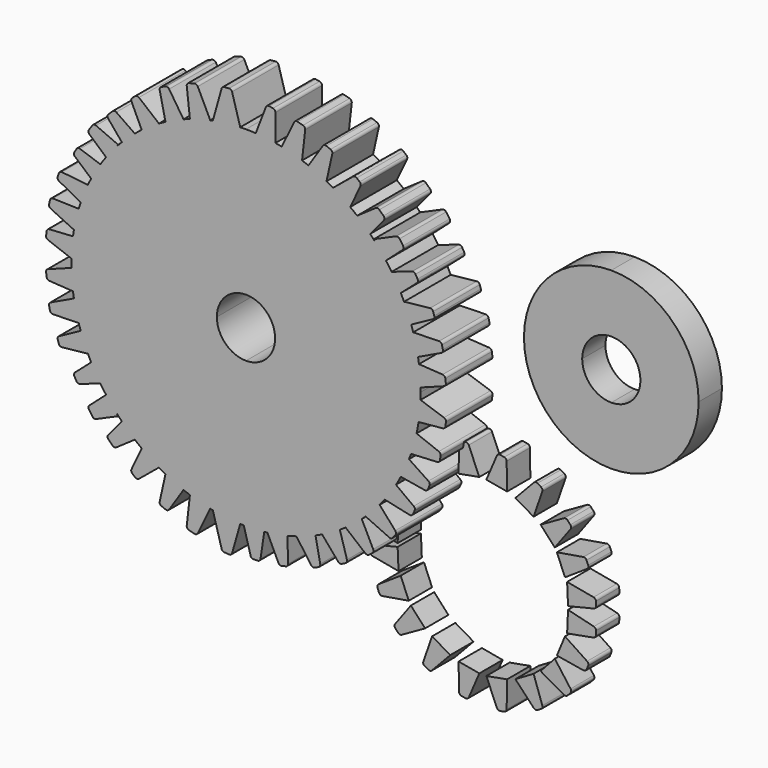
from build123d import *

# Parameters (mm, degrees)
F1_DEPTH = 12.7
F3_DEPTH = 6.35
F5_DEPTH = 12.7


with BuildPart() as f1:
    # F0 (on Front) → F1 (new body)
    with BuildSketch(Plane.XZ):
        with BuildLine():
            Line((-40.2337083757, 35.2117754519), (-8.4837083757, 35.2117754519))
            ThreePointArc((-8.4837083757, 35.2117754519), (-19.6429400125, 62.1525438151), (-46.5837083757, 73.3117754519))
            Line((-46.5837083757, 73.3117754519), (-46.5837083757, 41.5617754519))
            ThreePointArc((-46.5837083757, 41.5617754519), (-42.0935803152, 39.7019035124), (-40.2337083757, 35.2117754519))
        make_face()
        with BuildLine():
            ThreePointArc((-46.5837083757, -2.8882245481), (-19.6429400125, 8.2710070887), (-8.4837083757, 35.2117754519))
            Line((-8.4837083757, 35.2117754519), (-40.2337083757, 35.2117754519))
            ThreePointArc((-40.2337083757, 35.2117754519), (-42.0935803152, 30.7216473914), (-46.5837083757, 28.8617754519))
            Line((-46.5837083757, 28.8617754519), (-46.5837083757, -2.8882245481))
        make_face()
        with BuildLine():
            Line((-46.5837083757, 41.5617754519), (-46.5837083757, 73.3117754519))
            ThreePointArc((-46.5837083757, 73.3117754519), (-73.5244767389, 62.1525438151), (-84.6837083757, 35.2117754519))
            Line((-84.6837083757, 35.2117754519), (-52.9337083757, 35.2117754519))
            ThreePointArc((-52.9337083757, 35.2117754519), (-51.0738364362, 39.7019035124), (-46.5837083757, 41.5617754519))
        make_face()
        with BuildLine():
            ThreePointArc((-84.6837083757, 35.2117754519), (-73.5244767389, 8.2710070887), (-46.5837083757, -2.8882245481))
            Line((-46.5837083757, -2.8882245481), (-46.5837083757, 28.8617754519))
            ThreePointArc((-46.5837083757, 28.8617754519), (-51.0738364362, 30.7216473914), (-52.9337083757, 35.2117754519))
            Line((-52.9337083757, 35.2117754519), (-84.6837083757, 35.2117754519))
        make_face()
    extrude(amount=F1_DEPTH)

    # F4 (on Front) → F5 (join)
    with BuildSketch(Plane.XZ):
        with BuildLine():
            Line((-51.8969909596, 79.4116455872), (-53.8015343792, 72.633956309))
            Line((-53.8015343792, 72.633956309), (-47.8001066492, 73.1590132003))
            Line((-47.8001066492, 73.1590132003), (-49.617990034, 79.5071715805))
            ThreePointArc((-49.617990034, 79.5071715805), (-49.8686926776, 79.8556137836), (-50.2837967744, 79.9649406937))
            Line((-50.2837967744, 79.9649406937), (-51.3410119919, 79.8724463472))
            ThreePointArc((-51.3410119919, 79.8724463472), (-51.6908785069, 79.7287691696), (-51.8969909596, 79.4116455872))
        make_face()
        with BuildLine():
            Line((-42.2328064249, 79.0054519707), (-44.4691890873, 73.2130066024))
            Line((-44.4691890873, 73.2130066024), (-40.1563979685, 72.452545166))
            Line((-40.1563979685, 72.452545166), (-40.1633544982, 78.628976981))
            ThreePointArc((-40.1633544982, 78.628976981), (-40.3121458126, 79.0367057851), (-40.6880875027, 79.2536147027))
            Line((-40.6880875027, 79.2536147027), (-41.5301577643, 79.4020944094))
            ThreePointArc((-41.5301577643, 79.4020944094), (-41.9525783878, 79.3297196605), (-42.2328064249, 79.0054519707))
        make_face()
        with BuildLine():
            Line((-36.0689035478, 78.103844477), (-38.8663043489, 72.3492131525))
            Line((-38.8663043489, 72.3492131525), (-34.3722383724, 71.1606460637))
            Line((-34.3722383724, 71.1606460637), (-33.6627541723, 77.4364471221))
            ThreePointArc((-33.6627541723, 77.4364471221), (-33.7695873359, 77.8662411035), (-34.1313756691, 78.1216728815))
            Line((-34.1313756691, 78.1216728815), (-35.335446186, 78.4401191608))
            ThreePointArc((-35.335446186, 78.4401191608), (-35.7624505237, 78.4034506042), (-36.0689035478, 78.103844477))
        make_face()
        with BuildLine():
            Line((-29.8271216895, 75.5803222566), (-33.0810726733, 70.5999554881))
            Line((-33.0810726733, 70.5999554881), (-29.0387614156, 68.9628200449))
            Line((-29.0387614156, 68.9628200449), (-27.7608324195, 74.7250371239))
            ThreePointArc((-27.7608324195, 74.7250371239), (-27.8186671264, 75.1579330672), (-28.1424018291, 75.4510876225))
            Line((-28.1424018291, 75.4510876225), (-29.0571588688, 75.8215640841))
            ThreePointArc((-29.0571588688, 75.8215640841), (-29.485381743, 75.8389553876), (-29.8271216895, 75.5803222566))
        make_face()
        with BuildLine():
            Line((-23.2376398868, 71.822821528), (-27.7401155231, 68.1239195251))
            Line((-27.7401155231, 68.1239195251), (-24.0639013158, 65.3104154524))
            Line((-24.0639013158, 65.3104154524), (-21.6101830678, 70.5265202369))
            ThreePointArc((-21.6101830678, 70.5265202369), (-21.565222672, 70.9359992505), (-21.7809995875, 71.2869049679))
            Line((-21.7809995875, 71.2869049679), (-22.4307693654, 71.8222503924))
            ThreePointArc((-22.4307693654, 71.8222503924), (-22.8341022527, 71.9671637093), (-23.2376398868, 71.822821528))
        make_face()
        with BuildLine():
            Line((-18.299348504, 67.3945537621), (-22.639352635, 64.3854139528))
            Line((-22.639352635, 64.3854139528), (-19.8183730245, 61.6465695202))
            Line((-19.8183730245, 61.6465695202), (-16.5385630676, 65.5814843759))
            ThreePointArc((-16.5385630676, 65.5814843759), (-16.3922203601, 66.0214788509), (-16.5840087504, 66.4436500714))
            Line((-16.5840087504, 66.4436500714), (-17.495201454, 67.3283126382))
            ThreePointArc((-17.495201454, 67.3283126382), (-17.8854015688, 67.5055727798), (-18.299348504, 67.3945537621))
        make_face()
        with BuildLine():
            Line((-6.4277782702, 52.0293163314), (-12.2672549008, 51.3959517145))
            Line((-12.2672549008, 51.3959517145), (-10.990546413, 47.2971975058))
            Line((-10.990546413, 47.2971975058), (-5.8245082358, 50.0928984036))
            ThreePointArc((-5.8245082358, 50.0928984036), (-5.5385502609, 50.4120623727), (-5.5204638467, 50.8402101091))
            Line((-5.5204638467, 50.8402101091), (-5.7530367391, 51.5868638132))
            ThreePointArc((-5.7530367391, 51.5868638132), (-6.0110999701, 51.9290343209), (-6.4277782702, 52.0293163314))
        make_face()
        with BuildLine():
            Line((-4.4669738122, 46.3248511888), (-10.2619681871, 46.1824522754))
            Line((-10.2619681871, 46.1824522754), (-9.2668208617, 41.700486656))
            Line((-9.2668208617, 41.700486656), (-3.9791937156, 44.2206923841))
            ThreePointArc((-3.9791937156, 44.2206923841), (-3.6816644799, 44.5155571011), (-3.6325001912, 44.931551957))
            Line((-3.6325001912, 44.931551957), (-3.8314713048, 45.8276822761))
            ThreePointArc((-3.8314713048, 45.8276822761), (-4.0601073673, 46.1901775704), (-4.4669738122, 46.3248511888))
        make_face()
        with BuildLine():
            Line((-10.3613183438, 57.7898576628), (-15.3773872066, 56.073537705))
            Line((-15.3773872066, 56.073537705), (-13.6202546353, 52.1526247588))
            Line((-13.6202546353, 52.1526247588), (-9.2861122979, 55.9260926097))
            ThreePointArc((-9.2861122979, 55.9260926097), (-9.0767465829, 56.3004482758), (-9.1531520594, 56.7225126909))
            Line((-9.1531520594, 56.7225126909), (-9.6058187546, 57.506554406))
            ThreePointArc((-9.6058187546, 57.506554406), (-9.9327877718, 57.7836257854), (-10.3613183438, 57.7898576628))
        make_face()
        with BuildLine():
            Line((-3.6967090518, 40.1622607761), (-9.4820626067, 40.5254707725))
            Line((-9.4820626067, 40.5254707725), (-8.8813311598, 35.9738275811))
            Line((-8.8813311598, 35.9738275811), (-3.3941746293, 38.0235960943))
            ThreePointArc((-3.3941746293, 38.0235960943), (-3.0720784288, 38.2914073805), (-2.9868448844, 38.7015343003))
            Line((-2.9868448844, 38.7015343003), (-3.1069559492, 39.6115960482))
            ThreePointArc((-3.1069559492, 39.6115960482), (-3.3031284358, 39.9926388843), (-3.6967090518, 40.1622607761))
        make_face()
        with BuildLine():
            Line((-30.3894224423, -4.9122257304), (-31.535948209, 0.7700023469))
            Line((-31.535948209, 0.7700023469), (-35.7770171801, -0.9883116168))
            Line((-35.7770171801, -0.9883116168), (-32.3769122218, -5.7579786932))
            ThreePointArc((-32.3769122218, -5.7579786932), (-32.0348617529, -5.9997850705), (-31.6166495044, -5.9759656945))
            Line((-31.6166495044, -5.9759656945), (-30.7686843897, -5.6244060024))
            ThreePointArc((-30.7686843897, -5.6244060024), (-30.4513984491, -5.3362967882), (-30.3894224423, -4.9122257304))
        make_face()
        with BuildLine():
            Line((-37.4045271294, -7.1601327794), (-37.5469260428, -1.3651384045))
            Line((-37.5469260428, -1.3651384045), (-42.0288916622, -2.3602857299))
            Line((-42.0288916622, -2.3602857299), (-39.5086859341, -7.6479128759))
            ThreePointArc((-39.5086859341, -7.6479128759), (-39.2138212171, -7.9454421116), (-38.7978263612, -7.9946064003))
            Line((-38.7978263612, -7.9946064003), (-37.9016960421, -7.7956352867))
            ThreePointArc((-37.9016960421, -7.7956352867), (-37.5392007478, -7.5669992243), (-37.4045271294, -7.1601327794))
        make_face()
        with BuildLine():
            Line((-24.5531178016, -2.1839883726), (-26.1905195002, 3.3766908065))
            Line((-26.1905195002, 3.3766908065), (-30.262202764, 1.2554342421))
            Line((-30.262202764, 1.2554342421), (-26.4593323549, -3.199744138))
            ThreePointArc((-26.4593323549, -3.199744138), (-26.0975086768, -3.4108187063), (-25.6829638476, -3.3506403712))
            Line((-25.6829638476, -3.3506403712), (-24.8688659423, -2.9265134404))
            ThreePointArc((-24.8688659423, -2.9265134404), (-24.577897743, -2.6118472769), (-24.5531178016, -2.1839883726))
        make_face()
        with BuildLine():
            Line((-18.8384442582, 1.6800521382), (-21.4165719518, 6.8719202848))
            Line((-21.4165719518, 6.8719202848), (-25.058044861, 4.0758499952))
            Line((-25.058044861, 4.0758499952), (-20.5393149915, 0.3487173019))
            ThreePointArc((-20.5393149915, 0.3487173019), (-20.146335514, 0.2036794529), (-19.7485384105, 0.334928498))
            Line((-19.7485384105, 0.334928498), (-19.0204573502, 0.8939786054))
            ThreePointArc((-19.0204573502, 0.8939786054), (-18.7885508175, 1.2543903804), (-18.8384442582, 1.6800521382))
        make_face()
        with BuildLine():
            Line((-14.0267707257, 6.8227043457), (-17.8608052044, 11.1703953274))
            Line((-17.8608052044, 11.1703953274), (-20.6545216907, 7.5271162815))
            Line((-20.6545216907, 7.5271162815), (-15.3251108831, 5.0965159049))
            ThreePointArc((-15.3251108831, 5.0965159049), (-14.907983299, 5.0581306738), (-14.5577105556, 5.2878649827))
            Line((-14.5577105556, 5.2878649827), (-13.9991310708, 6.0163071644))
            ThreePointArc((-13.9991310708, 6.0163071644), (-13.8684079931, 6.4244600333), (-14.0267707257, 6.8227043457))
        make_face()
        with BuildLine():
            Line((-9.998777359, 12.8348904358), (-14.6633019393, 16.2764667746))
            Line((-14.6633019393, 16.2764667746), (-16.6260565576, 12.1260537445))
            Line((-16.6260565576, 12.1260537445), (-10.9039764419, 10.8737610881))
            ThreePointArc((-10.9039764419, 10.8737610881), (-10.4881326431, 10.9241870969), (-10.1941718563, 11.2226094541))
            Line((-10.1941718563, 11.2226094541), (-9.8017360208, 12.0524486963))
            ThreePointArc((-9.8017360208, 12.0524486963), (-9.7600076851, 12.4789883), (-9.998777359, 12.8348904358))
        make_face()
        with BuildLine():
            Line((-6.7800339635, 18.7066511832), (-11.6086921136, 21.9138770445))
            Line((-11.6086921136, 21.9138770445), (-13.3642650154, 17.6716726884))
            Line((-13.3642650154, 17.6716726884), (-7.5873638089, 16.7032460274))
            ThreePointArc((-7.5873638089, 16.7032460274), (-7.1745146737, 16.7741293044), (-6.8956367991, 17.0866928635))
            Line((-6.8956367991, 17.0866928635), (-6.5446251586, 17.9348849886))
            ThreePointArc((-6.5446251586, 17.9348849886), (-6.5239940975, 18.3629640079), (-6.7800339635, 18.7066511832))
        make_face()
        with BuildLine():
            Line((-4.5182707136, 25.1217887225), (-9.9243117756, 27.2139066187))
            Line((-9.9243117756, 27.2139066187), (-10.7251306009, 22.6931740209))
            Line((-10.7251306009, 22.6931740209), (-4.8752228248, 22.9915307831))
            ThreePointArc((-4.8752228248, 22.9915307831), (-4.4873252593, 23.149658346), (-4.2823016206, 23.5149447473))
            Line((-4.2823016206, 23.5149447473), (-4.1221848124, 24.418826189))
            ThreePointArc((-4.1221848124, 24.418826189), (-4.1942250323, 24.8413039922), (-4.5182707136, 25.1217887225))
        make_face()
        with BuildLine():
            Line((-3.3938642901, 31.9966780583), (-8.8880810385, 33.8448716568))
            Line((-8.8880810385, 33.8448716568), (-9.4858709636, 29.2928412068))
            Line((-9.4858709636, 29.2928412068), (-3.6551656288, 29.852584938))
            ThreePointArc((-3.6551656288, 29.852584938), (-3.2747299287, 30.0279061449), (-3.0862519892, 30.4019982642))
            Line((-3.0862519892, 30.4019982642), (-2.9667290562, 31.3121374411))
            ThreePointArc((-2.9667290562, 31.3121374411), (-3.0575959844, 31.7309697331), (-3.3938642901, 31.9966780583))
        make_face()
        with BuildLine():
            Line((-13.8675008132, 63.3961231942), (-18.6919855671, 61.2844998724))
            Line((-18.6919855671, 61.2844998724), (-16.2907256709, 57.8230131868))
            Line((-16.2907256709, 57.8230131868), (-12.4314796339, 61.2432696639))
            ThreePointArc((-12.4314796339, 61.2432696639), (-12.2221835139, 61.6427507415), (-12.3308996786, 62.0804387499))
            Line((-12.3308996786, 62.0804387499), (-13.0911386736, 63.1763455957))
            ThreePointArc((-13.0911386736, 63.1763455957), (-13.4399256416, 63.4253936601), (-13.8675008132, 63.3961231942))
        make_face()
        with BuildLine():
            Line((-58.795178379, 71.1606460637), (-54.3011124025, 72.3492131525))
            Line((-54.3011124025, 72.3492131525), (-57.0985132036, 78.103844477))
            ThreePointArc((-57.0985132036, 78.103844477), (-57.4049662277, 78.4034506042), (-57.8319705654, 78.4401191608))
            Line((-57.8319705654, 78.4401191608), (-59.0360410823, 78.1216728815))
            ThreePointArc((-59.0360410823, 78.1216728815), (-59.3978294155, 77.8662411035), (-59.5046625791, 77.4364471221))
            Line((-59.5046625791, 77.4364471221), (-58.795178379, 71.1606460637))
        make_face()
        with BuildLine():
            ThreePointArc((-65.0250149222, 75.4510876225), (-65.348749625, 75.1579330672), (-65.4065843319, 74.7250371239))
            Line((-65.4065843319, 74.7250371239), (-64.1286553358, 68.9628200449))
            Line((-64.1286553358, 68.9628200449), (-60.0863440781, 70.5999554881))
            Line((-60.0863440781, 70.5999554881), (-63.3402950619, 75.5803222566))
            ThreePointArc((-63.3402950619, 75.5803222566), (-63.6820350084, 75.8389553876), (-64.1102578826, 75.8215640841))
            Line((-64.1102578826, 75.8215640841), (-65.0250149222, 75.4510876225))
        make_face()
        with BuildLine():
            Line((-69.1035154356, 65.3104154524), (-65.4273012282, 68.1239195251))
            Line((-65.4273012282, 68.1239195251), (-69.9297768646, 71.822821528))
            ThreePointArc((-69.9297768646, 71.822821528), (-70.3333144987, 71.9671637093), (-70.736647386, 71.8222503924))
            Line((-70.736647386, 71.8222503924), (-71.3864171639, 71.2869049679))
            ThreePointArc((-71.3864171639, 71.2869049679), (-71.6021940794, 70.9359992505), (-71.5572336836, 70.5265202369))
            Line((-71.5572336836, 70.5265202369), (-69.1035154356, 65.3104154524))
        make_face()
        with BuildLine():
            ThreePointArc((-76.583408001, 66.4436500714), (-76.7751963913, 66.0214788509), (-76.6288536838, 65.5814843759))
            Line((-76.6288536838, 65.5814843759), (-73.3490437269, 61.6465695202))
            Line((-73.3490437269, 61.6465695202), (-70.5280641164, 64.3854139528))
            Line((-70.5280641164, 64.3854139528), (-74.8680682474, 67.3945537621))
            ThreePointArc((-74.8680682474, 67.3945537621), (-75.2820151826, 67.5055727798), (-75.6722152974, 67.3283126382))
            Line((-75.6722152974, 67.3283126382), (-76.583408001, 66.4436500714))
        make_face()
        with BuildLine():
            Line((-76.8766910805, 57.8230131868), (-74.4754311843, 61.2844998724))
            Line((-74.4754311843, 61.2844998724), (-79.2999159382, 63.3961231942))
            ThreePointArc((-79.2999159382, 63.3961231942), (-79.7274911097, 63.4253936601), (-80.0762780778, 63.1763455957))
            Line((-80.0762780778, 63.1763455957), (-80.8365170728, 62.0804387499))
            ThreePointArc((-80.8365170728, 62.0804387499), (-80.9452332375, 61.6427507415), (-80.7359371175, 61.2432696639))
            Line((-80.7359371175, 61.2432696639), (-76.8766910805, 57.8230131868))
        make_face()
        with BuildLine():
            ThreePointArc((-84.014264692, 56.7225126909), (-84.0906701685, 56.3004482758), (-83.8813044535, 55.9260926097))
            Line((-83.8813044535, 55.9260926097), (-79.5471621161, 52.1526247588))
            Line((-79.5471621161, 52.1526247588), (-77.7900295448, 56.073537705))
            Line((-77.7900295448, 56.073537705), (-82.8060984076, 57.7898576628))
            ThreePointArc((-82.8060984076, 57.7898576628), (-83.2346289796, 57.7836257854), (-83.5615979968, 57.506554406))
            Line((-83.5615979968, 57.506554406), (-84.014264692, 56.7225126909))
        make_face()
        with BuildLine():
            ThreePointArc((-87.6469529046, 50.8402101091), (-87.6288664905, 50.4120623727), (-87.3429085156, 50.0928984036))
            Line((-87.3429085156, 50.0928984036), (-82.1768703384, 47.2971975058))
            Line((-82.1768703384, 47.2971975058), (-80.9001618506, 51.3959517145))
            Line((-80.9001618506, 51.3959517145), (-86.7396384812, 52.0293163314))
            ThreePointArc((-86.7396384812, 52.0293163314), (-87.1563167813, 51.9290343209), (-87.4143800123, 51.5868638132))
            Line((-87.4143800123, 51.5868638132), (-87.6469529046, 50.8402101091))
        make_face()
        with BuildLine():
            ThreePointArc((-89.5349165602, 44.931551957), (-89.4857522714, 44.5155571011), (-89.1882230357, 44.2206923841))
            Line((-89.1882230357, 44.2206923841), (-83.9005958897, 41.700486656))
            Line((-83.9005958897, 41.700486656), (-82.9054485643, 46.1824522754))
            Line((-82.9054485643, 46.1824522754), (-88.7004429392, 46.3248511888))
            ThreePointArc((-88.7004429392, 46.3248511888), (-89.1073093841, 46.1901775704), (-89.3359454466, 45.8276822761))
            Line((-89.3359454466, 45.8276822761), (-89.5349165602, 44.931551957))
        make_face()
        with BuildLine():
            Line((-84.2860855916, 35.9738275811), (-83.6853541447, 40.5254707725))
            Line((-83.6853541447, 40.5254707725), (-89.4707076996, 40.1622607761))
            ThreePointArc((-89.4707076996, 40.1622607761), (-89.8642883155, 39.9926388843), (-90.0604608022, 39.6115960482))
            Line((-90.0604608022, 39.6115960482), (-90.180571867, 38.7015343003))
            ThreePointArc((-90.180571867, 38.7015343003), (-90.0953383226, 38.2914073805), (-89.7732421221, 38.0235960943))
            Line((-89.7732421221, 38.0235960943), (-84.2860855916, 35.9738275811))
        make_face()
        with BuildLine():
            Line((-84.2860855916, 34.4497233226), (-89.7732421221, 32.3999548095))
            ThreePointArc((-89.7732421221, 32.3999548095), (-90.0953383226, 32.1321435233), (-90.180571867, 31.7220166035))
            Line((-90.180571867, 31.7220166035), (-90.0604608022, 30.8119548556))
            ThreePointArc((-90.0604608022, 30.8119548556), (-89.8642883155, 30.4309120195), (-89.4707076996, 30.2612901277))
            Line((-89.4707076996, 30.2612901277), (-83.6853541447, 29.8980801313))
            Line((-83.6853541447, 29.8980801313), (-84.2860855916, 34.4497233226))
        make_face()
        with BuildLine():
            Line((-83.9005958897, 28.7230642478), (-89.1882230357, 26.2028585197))
            ThreePointArc((-89.1882230357, 26.2028585197), (-89.4857522714, 25.9079938027), (-89.5349165602, 25.4919989468))
            Line((-89.5349165602, 25.4919989468), (-89.3359454466, 24.5958686277))
            ThreePointArc((-89.3359454466, 24.5958686277), (-89.1073093841, 24.2333733334), (-88.7004429392, 24.098699715))
            Line((-88.7004429392, 24.098699715), (-82.9054485643, 24.2410986284))
            Line((-82.9054485643, 24.2410986284), (-83.9005958897, 28.7230642478))
        make_face()
        with BuildLine():
            Line((-82.1768703384, 23.126353398), (-87.3429085156, 20.3306525002))
            ThreePointArc((-87.3429085156, 20.3306525002), (-87.6288664905, 20.0114885311), (-87.6469529046, 19.5833407947))
            Line((-87.6469529046, 19.5833407947), (-87.4143800123, 18.8366870906))
            ThreePointArc((-87.4143800123, 18.8366870906), (-87.1563167813, 18.4945165829), (-86.7396384812, 18.3942345724))
            Line((-86.7396384812, 18.3942345724), (-80.9001618506, 19.0275991893))
            Line((-80.9001618506, 19.0275991893), (-82.1768703384, 23.126353398))
        make_face()
        with BuildLine():
            Line((-82.8060984076, 12.633693241), (-77.7900295448, 14.3500131988))
            Line((-77.7900295448, 14.3500131988), (-79.5471621161, 18.270926145))
            Line((-79.5471621161, 18.270926145), (-83.8813044535, 14.497458294))
            ThreePointArc((-83.8813044535, 14.497458294), (-84.0906701685, 14.123102628), (-84.014264692, 13.7010382129))
            Line((-84.014264692, 13.7010382129), (-83.5615979968, 12.9169964978))
            ThreePointArc((-83.5615979968, 12.9169964978), (-83.2346289796, 12.6399251184), (-82.8060984076, 12.633693241))
        make_face()
        with BuildLine():
            Line((-79.2999159382, 7.0274277096), (-74.4754311843, 9.1390510314))
            Line((-74.4754311843, 9.1390510314), (-76.8766910805, 12.600537717))
            Line((-76.8766910805, 12.600537717), (-80.7359371175, 9.1802812399))
            ThreePointArc((-80.7359371175, 9.1802812399), (-80.9452332375, 8.7808001623), (-80.8365170728, 8.3431121539))
            Line((-80.8365170728, 8.3431121539), (-80.0762780778, 7.2472053081))
            ThreePointArc((-80.0762780778, 7.2472053081), (-79.7274911097, 6.9981572437), (-79.2999159382, 7.0274277096))
        make_face()
        with BuildLine():
            Line((-73.3490437269, 8.7769813836), (-76.6288536838, 4.8420665279))
            ThreePointArc((-76.6288536838, 4.8420665279), (-76.7751963913, 4.4020720529), (-76.583408001, 3.9799008324))
            Line((-76.583408001, 3.9799008324), (-75.6722152974, 3.0952382656))
            ThreePointArc((-75.6722152974, 3.0952382656), (-75.2820151826, 2.917978124), (-74.8680682474, 3.0289971417))
            Line((-74.8680682474, 3.0289971417), (-70.5280641164, 6.038136951))
            Line((-70.5280641164, 6.038136951), (-73.3490437269, 8.7769813836))
        make_face()
        with BuildLine():
            Line((-69.9297768646, -1.3992706242), (-65.4273012282, 2.2996313787))
            Line((-65.4273012282, 2.2996313787), (-69.1035154356, 5.1131354514))
            Line((-69.1035154356, 5.1131354514), (-71.5572336836, -0.1029693331))
            ThreePointArc((-71.5572336836, -0.1029693331), (-71.6021940794, -0.5124483467), (-71.3864171639, -0.8633540641))
            Line((-71.3864171639, -0.8633540641), (-70.736647386, -1.3986994886))
            ThreePointArc((-70.736647386, -1.3986994886), (-70.3333144987, -1.5436128055), (-69.9297768646, -1.3992706242))
        make_face()
        with BuildLine():
            Line((-64.1286553358, 1.4607308589), (-65.4065843319, -4.3014862201))
            ThreePointArc((-65.4065843319, -4.3014862201), (-65.348749625, -4.7343821634), (-65.0250149222, -5.0275367187))
            Line((-65.0250149222, -5.0275367187), (-64.1102578826, -5.3980131803))
            ThreePointArc((-64.1102578826, -5.3980131803), (-63.6820350084, -5.4154044838), (-63.3402950619, -5.1567713528))
            Line((-63.3402950619, -5.1567713528), (-60.0863440781, -0.1764045843))
            Line((-60.0863440781, -0.1764045843), (-64.1286553358, 1.4607308589))
        make_face()
        with BuildLine():
            Line((-58.795178379, -0.7370951599), (-59.5046625791, -7.0128962183))
            ThreePointArc((-59.5046625791, -7.0128962183), (-59.3978294155, -7.4426901997), (-59.0360410823, -7.6981219777))
            Line((-59.0360410823, -7.6981219777), (-57.8319705654, -8.016568257))
            ThreePointArc((-57.8319705654, -8.016568257), (-57.4049662277, -7.9798997004), (-57.0985132036, -7.6802935732))
            Line((-57.0985132036, -7.6802935732), (-54.3011124025, -1.9256622487))
            Line((-54.3011124025, -1.9256622487), (-58.795178379, -0.7370951599))
        make_face()
        with BuildLine():
            Line((-47.8001066492, -2.7354622965), (-53.8015343792, -2.2104054052))
            Line((-53.8015343792, -2.2104054052), (-51.8969909596, -8.9880946834))
            ThreePointArc((-51.8969909596, -8.9880946834), (-51.6908785069, -9.3052182658), (-51.3410119919, -9.4488954434))
            Line((-51.3410119919, -9.4488954434), (-50.2837967744, -9.5413897899))
            ThreePointArc((-50.2837967744, -9.5413897899), (-49.8686926776, -9.4320628798), (-49.617990034, -9.0836206767))
            Line((-49.617990034, -9.0836206767), (-47.8001066492, -2.7354622965))
        make_face()
        with BuildLine():
            Line((-43.4169813458, -8.1469004872), (-42.550926687, -2.4152177863))
            Line((-42.550926687, -2.4152177863), (-47.1376066972, -2.6169614256))
            Line((-47.1376066972, -2.6169614256), (-45.5738753751, -8.2618867661))
            ThreePointArc((-45.5738753751, -8.2618867661), (-45.3351557253, -8.6060985849), (-44.9340180551, -8.7267527062))
            Line((-44.9340180551, -8.7267527062), (-44.0169509979, -8.6864158078))
            ThreePointArc((-44.0169509979, -8.6864158078), (-43.620260586, -8.5241998881), (-43.4169813458, -8.1469004872))
        make_face()
    extrude(amount=F5_DEPTH)


with BuildPart() as f3:
    # F2 (on Front) → F3 (new body)
    with BuildSketch(Plane.XZ):
        with BuildLine():
            Line((34.3702440917, 48.854034394), (47.0702440917, 48.854034394))
            ThreePointArc((47.0702440917, 48.854034394), (41.4906282734, 62.3244185756), (28.0202440917, 67.904034394))
            Line((28.0202440917, 67.904034394), (28.0202440917, 55.204034394))
            ThreePointArc((28.0202440917, 55.204034394), (32.5103721523, 53.3441624546), (34.3702440917, 48.854034394))
        make_face()
        with BuildLine():
            ThreePointArc((28.0202440917, 29.804034394), (41.4906282734, 35.3836502124), (47.0702440917, 48.854034394))
            Line((47.0702440917, 48.854034394), (34.3702440917, 48.854034394))
            ThreePointArc((34.3702440917, 48.854034394), (32.5103721523, 44.3639063335), (28.0202440917, 42.504034394))
            Line((28.0202440917, 42.504034394), (28.0202440917, 29.804034394))
        make_face()
        with BuildLine():
            Line((28.0202440917, 55.204034394), (28.0202440917, 67.904034394))
            ThreePointArc((28.0202440917, 67.904034394), (14.5498599101, 62.3244185756), (8.9702440917, 48.854034394))
            Line((8.9702440917, 48.854034394), (21.6702440917, 48.854034394))
            ThreePointArc((21.6702440917, 48.854034394), (23.5301160312, 53.3441624546), (28.0202440917, 55.204034394))
        make_face()
        with BuildLine():
            ThreePointArc((8.9702440917, 48.854034394), (14.5498599101, 35.3836502124), (28.0202440917, 29.804034394))
            Line((28.0202440917, 29.804034394), (28.0202440917, 42.504034394))
            ThreePointArc((28.0202440917, 42.504034394), (23.5301160312, 44.3639063335), (21.6702440917, 48.854034394))
            Line((21.6702440917, 48.854034394), (8.9702440917, 48.854034394))
        make_face()
    extrude(amount=F3_DEPTH)


with BuildPart() as f3b:
    # F2 (on Front) → F3, piece 2 (new body)
    with BuildSketch(Plane.XZ):
        with BuildLine():
            Line((-5.1978806635, 23.8259554301), (-5.2834348379, 18.0298431349))
            Line((-5.2834348379, 18.0298431349), (-0.7658083537, 18.848002631))
            Line((-0.7658083537, 18.848002631), (-3.076170687, 24.230628722))
            ThreePointArc((-3.076170687, 24.230628722), (-3.3591093906, 24.5395211586), (-3.7728495885, 24.6050031876))
            Line((-3.7728495885, 24.6050031876), (-4.6761099896, 24.441419262))
            ThreePointArc((-4.6761099896, 24.441419262), (-5.0473143261, 24.2272122874), (-5.1978806635, 23.8259554301))
        make_face()
    extrude(amount=F3_DEPTH)


with BuildPart() as f3c:
    # F2 (on Front) → F3, piece 3 (new body)
    with BuildSketch(Plane.XZ):
        with BuildLine():
            Line((-12.976613467, 20.5542184263), (-11.067678728, 15.0808094868))
            Line((-11.067678728, 15.0808094868), (-7.1052629114, 17.3997736757))
            Line((-7.1052629114, 17.3997736757), (-11.1226685733, 21.6625063081))
            ThreePointArc((-11.1226685733, 21.6625063081), (-11.4944364852, 21.8555282424), (-11.905519525, 21.7750323927))
            Line((-11.905519525, 21.7750323927), (-12.6977703479, 21.3113755298))
            ThreePointArc((-12.6977703479, 21.3113755298), (-12.97290876, 20.9827782968), (-12.976613467, 20.5542184263))
        make_face()
    extrude(amount=F3_DEPTH)


with BuildPart() as f3d:
    # F2 (on Front) → F3, piece 4 (new body)
    with BuildSketch(Plane.XZ):
        with BuildLine():
            Line((-24.2185268411, 1.7212534059), (-18.5841365603, 0.3589452835))
            Line((-18.5841365603, 0.3589452835), (-18.3853570011, 4.9457547083))
            Line((-18.3853570011, 4.9457547083), (-24.1450898613, 3.8799615168))
            ThreePointArc((-24.1450898613, 3.8799615168), (-24.5087976386, 3.672150304), (-24.6639540862, 3.2830547834))
            Line((-24.6639540862, 3.2830547834), (-24.7036983424, 2.3659618508))
            ThreePointArc((-24.7036983424, 2.3659618508), (-24.5766735507, 1.9566429168), (-24.2185268411, 1.7212534059))
        make_face()
    extrude(amount=F3_DEPTH)


with BuildPart() as f3e:
    # F2 (on Front) → F3, piece 5 (new body)
    with BuildSketch(Plane.XZ):
        with BuildLine():
            Line((-22.7420120578, 8.875056106), (-17.9133539077, 5.6678302448))
            Line((-17.9133539077, 5.6678302448), (-16.1577810059, 9.9100346009))
            Line((-16.1577810059, 9.9100346009), (-21.9346822124, 10.8784612618))
            ThreePointArc((-21.9346822124, 10.8784612618), (-22.3475313476, 10.8075779848), (-22.6264092222, 10.4950144257))
            Line((-22.6264092222, 10.4950144257), (-22.9774208627, 9.6468223006))
            ThreePointArc((-22.9774208627, 9.6468223006), (-22.9980519238, 9.2187432813), (-22.7420120578, 8.875056106))
        make_face()
    extrude(amount=F3_DEPTH)


with BuildPart() as f3f:
    # F2 (on Front) → F3, piece 6 (new body)
    with BuildSketch(Plane.XZ):
        with BuildLine():
            Line((-19.1367242409, 15.3386047249), (-15.6962056577, 10.6732998973))
            Line((-15.6962056577, 10.6732998973), (-12.5955874147, 14.0592267311))
            Line((-12.5955874147, 14.0592267311), (-17.6928774241, 16.9450666968))
            ThreePointArc((-17.6928774241, 16.9450666968), (-18.1050722185, 17.0196609249), (-18.4740347327, 16.8213291055))
            Line((-18.4740347327, 16.8213291055), (-19.0939765732, 16.1443422761))
            ThreePointArc((-19.0939765732, 16.1443422761), (-19.2597750767, 15.749135819), (-19.1367242409, 15.3386047249))
        make_face()
    extrude(amount=F3_DEPTH)


with BuildPart() as f3g:
    # F2 (on Front) → F3, piece 7 (new body)
    with BuildSketch(Plane.XZ):
        with BuildLine():
            Line((0.7658083537, 18.848002631), (5.2834348379, 18.0298431349))
            Line((5.2834348379, 18.0298431349), (5.1978806635, 23.8259554301))
            ThreePointArc((5.1978806635, 23.8259554301), (5.0473143261, 24.2272122874), (4.6761099896, 24.441419262))
            Line((4.6761099896, 24.441419262), (3.7728495885, 24.6050031876))
            ThreePointArc((3.7728495885, 24.6050031876), (3.3591093906, 24.5395211586), (3.076170687, 24.230628722))
            Line((3.076170687, 24.230628722), (0.7658083537, 18.848002631))
        make_face()
    extrude(amount=F3_DEPTH)


with BuildPart() as f3h:
    # F2 (on Front) → F3, piece 8 (new body)
    with BuildSketch(Plane.XZ):
        with BuildLine():
            Line((7.1052629114, 17.3997736757), (11.067678728, 15.0808094868))
            Line((11.067678728, 15.0808094868), (12.976613467, 20.5542184263))
            ThreePointArc((12.976613467, 20.5542184263), (12.97290876, 20.9827782968), (12.6977703479, 21.3113755298))
            Line((12.6977703479, 21.3113755298), (11.905519525, 21.7750323927))
            ThreePointArc((11.905519525, 21.7750323927), (11.4944364852, 21.8555282424), (11.1226685733, 21.6625063081))
            Line((11.1226685733, 21.6625063081), (7.1052629114, 17.3997736757))
        make_face()
    extrude(amount=F3_DEPTH)


with BuildPart() as f3i:
    # F2 (on Front) → F3, piece 9 (new body)
    with BuildSketch(Plane.XZ):
        with BuildLine():
            Line((12.5955874147, 14.0592267311), (15.6962056577, 10.6732998973))
            Line((15.6962056577, 10.6732998973), (19.1367242409, 15.3386047249))
            ThreePointArc((19.1367242409, 15.3386047249), (19.2597750767, 15.749135819), (19.0939765732, 16.1443422761))
            Line((19.0939765732, 16.1443422761), (18.4740347327, 16.8213291055))
            ThreePointArc((18.4740347327, 16.8213291055), (18.1050722185, 17.0196609249), (17.6928774241, 16.9450666968))
            Line((17.6928774241, 16.9450666968), (12.5955874147, 14.0592267311))
        make_face()
    extrude(amount=F3_DEPTH)


with BuildPart() as f3j:
    # F2 (on Front) → F3, piece 10 (new body)
    with BuildSketch(Plane.XZ):
        with BuildLine():
            Line((16.1577810059, 9.9100346009), (17.9133539077, 5.6678302448))
            Line((17.9133539077, 5.6678302448), (22.7420120578, 8.875056106))
            ThreePointArc((22.7420120578, 8.875056106), (22.9980519238, 9.2187432813), (22.9774208627, 9.6468223006))
            Line((22.9774208627, 9.6468223006), (22.6264092222, 10.4950144257))
            ThreePointArc((22.6264092222, 10.4950144257), (22.3475313476, 10.8075779848), (21.9346822124, 10.8784612618))
            Line((21.9346822124, 10.8784612618), (16.1577810059, 9.9100346009))
        make_face()
    extrude(amount=F3_DEPTH)


with BuildPart() as f3k:
    # F2 (on Front) → F3, piece 11 (new body)
    with BuildSketch(Plane.XZ):
        with BuildLine():
            Line((18.3853570011, 4.9457547083), (18.5841365603, 0.3589452835))
            Line((18.5841365603, 0.3589452835), (24.2185268411, 1.7212534059))
            ThreePointArc((24.2185268411, 1.7212534059), (24.5766735507, 1.9566429168), (24.7036983424, 2.3659618508))
            Line((24.7036983424, 2.3659618508), (24.6639540862, 3.2830547834))
            ThreePointArc((24.6639540862, 3.2830547834), (24.5087976386, 3.672150304), (24.1450898613, 3.8799615168))
            Line((24.1450898613, 3.8799615168), (18.3853570011, 4.9457547083))
        make_face()
    extrude(amount=F3_DEPTH)


with BuildPart() as f3l:
    # F2 (on Front) → F3, piece 12 (new body)
    with BuildSketch(Plane.XZ):
        with BuildLine():
            Line((0.7658083537, -18.848002631), (3.076170687, -24.230628722))
            ThreePointArc((3.076170687, -24.230628722), (3.3591093906, -24.5395211586), (3.7728495885, -24.6050031876))
            Line((3.7728495885, -24.6050031876), (4.6761099896, -24.441419262))
            ThreePointArc((4.6761099896, -24.441419262), (5.0473143261, -24.2272122874), (5.1978806635, -23.8259554301))
            Line((5.1978806635, -23.8259554301), (5.2834348379, -18.0298431349))
            Line((5.2834348379, -18.0298431349), (0.7658083537, -18.848002631))
        make_face()
    extrude(amount=F3_DEPTH)


with BuildPart() as f3m:
    # F2 (on Front) → F3, piece 13 (new body)
    with BuildSketch(Plane.XZ):
        with BuildLine():
            Line((7.1052629114, -17.3997736757), (11.1226685733, -21.6625063081))
            ThreePointArc((11.1226685733, -21.6625063081), (11.4944364852, -21.8555282424), (11.905519525, -21.7750323927))
            Line((11.905519525, -21.7750323927), (12.6977703479, -21.3113755298))
            ThreePointArc((12.6977703479, -21.3113755298), (12.97290876, -20.9827782968), (12.976613467, -20.5542184263))
            Line((12.976613467, -20.5542184263), (11.067678728, -15.0808094868))
            Line((11.067678728, -15.0808094868), (7.1052629114, -17.3997736757))
        make_face()
    extrude(amount=F3_DEPTH)


with BuildPart() as f3n:
    # F2 (on Front) → F3, piece 14 (new body)
    with BuildSketch(Plane.XZ):
        with BuildLine():
            Line((12.5955874147, -14.0592267311), (17.6928774241, -16.9450666968))
            ThreePointArc((17.6928774241, -16.9450666968), (18.1050722185, -17.0196609249), (18.4740347327, -16.8213291055))
            Line((18.4740347327, -16.8213291055), (19.0939765732, -16.1443422761))
            ThreePointArc((19.0939765732, -16.1443422761), (19.2597750767, -15.749135819), (19.1367242409, -15.3386047249))
            Line((19.1367242409, -15.3386047249), (15.6962056577, -10.6732998973))
            Line((15.6962056577, -10.6732998973), (12.5955874147, -14.0592267311))
        make_face()
    extrude(amount=F3_DEPTH)


with BuildPart() as f3o:
    # F2 (on Front) → F3, piece 15 (new body)
    with BuildSketch(Plane.XZ):
        with BuildLine():
            Line((16.1577810059, -9.9100346009), (21.9346822124, -10.8784612618))
            ThreePointArc((21.9346822124, -10.8784612618), (22.3475313476, -10.8075779848), (22.6264092222, -10.4950144257))
            Line((22.6264092222, -10.4950144257), (22.9774208627, -9.6468223006))
            ThreePointArc((22.9774208627, -9.6468223006), (22.9980519238, -9.2187432813), (22.7420120578, -8.875056106))
            Line((22.7420120578, -8.875056106), (17.9133539077, -5.6678302448))
            Line((17.9133539077, -5.6678302448), (16.1577810059, -9.9100346009))
        make_face()
    extrude(amount=F3_DEPTH)


with BuildPart() as f3p:
    # F2 (on Front) → F3, piece 16 (new body)
    with BuildSketch(Plane.XZ):
        with BuildLine():
            Line((24.2185268411, -1.7212534059), (18.5841365603, -0.3589452835))
            Line((18.5841365603, -0.3589452835), (18.3853570011, -4.9457547083))
            Line((18.3853570011, -4.9457547083), (24.1450898613, -3.8799615168))
            ThreePointArc((24.1450898613, -3.8799615168), (24.5087976386, -3.672150304), (24.6639540862, -3.2830547834))
            Line((24.6639540862, -3.2830547834), (24.7036983424, -2.3659618508))
            ThreePointArc((24.7036983424, -2.3659618508), (24.5766735507, -1.9566429168), (24.2185268411, -1.7212534059))
        make_face()
    extrude(amount=F3_DEPTH)


with BuildPart() as f3q:
    # F2 (on Front) → F3, piece 17 (new body)
    with BuildSketch(Plane.XZ):
        with BuildLine():
            Line((-18.3853570011, -4.9457547083), (-18.5841365603, -0.3589452835))
            Line((-18.5841365603, -0.3589452835), (-24.2185268411, -1.7212534059))
            ThreePointArc((-24.2185268411, -1.7212534059), (-24.5766735507, -1.9566429168), (-24.7036983424, -2.3659618508))
            Line((-24.7036983424, -2.3659618508), (-24.6639540862, -3.2830547834))
            ThreePointArc((-24.6639540862, -3.2830547834), (-24.5087976386, -3.672150304), (-24.1450898613, -3.8799615168))
            Line((-24.1450898613, -3.8799615168), (-18.3853570011, -4.9457547083))
        make_face()
    extrude(amount=F3_DEPTH)


with BuildPart() as f3r:
    # F2 (on Front) → F3, piece 18 (new body)
    with BuildSketch(Plane.XZ):
        with BuildLine():
            Line((-16.1577810059, -9.9100346009), (-17.9133539077, -5.6678302448))
            Line((-17.9133539077, -5.6678302448), (-22.7420120578, -8.875056106))
            ThreePointArc((-22.7420120578, -8.875056106), (-22.9980519238, -9.2187432813), (-22.9774208627, -9.6468223006))
            Line((-22.9774208627, -9.6468223006), (-22.6264092222, -10.4950144257))
            ThreePointArc((-22.6264092222, -10.4950144257), (-22.3475313476, -10.8075779848), (-21.9346822124, -10.8784612618))
            Line((-21.9346822124, -10.8784612618), (-16.1577810059, -9.9100346009))
        make_face()
    extrude(amount=F3_DEPTH)


with BuildPart() as f3s:
    # F2 (on Front) → F3, piece 19 (new body)
    with BuildSketch(Plane.XZ):
        with BuildLine():
            Line((-12.5955874147, -14.0592267311), (-15.6962056577, -10.6732998973))
            Line((-15.6962056577, -10.6732998973), (-19.1367242409, -15.3386047249))
            ThreePointArc((-19.1367242409, -15.3386047249), (-19.2597750767, -15.749135819), (-19.0939765732, -16.1443422761))
            Line((-19.0939765732, -16.1443422761), (-18.4740347327, -16.8213291055))
            ThreePointArc((-18.4740347327, -16.8213291055), (-18.1050722185, -17.0196609249), (-17.6928774241, -16.9450666968))
            Line((-17.6928774241, -16.9450666968), (-12.5955874147, -14.0592267311))
        make_face()
    extrude(amount=F3_DEPTH)


with BuildPart() as f3t:
    # F2 (on Front) → F3, piece 20 (new body)
    with BuildSketch(Plane.XZ):
        with BuildLine():
            Line((-7.1052629114, -17.3997736757), (-11.067678728, -15.0808094868))
            Line((-11.067678728, -15.0808094868), (-12.976613467, -20.5542184263))
            ThreePointArc((-12.976613467, -20.5542184263), (-12.97290876, -20.9827782968), (-12.6977703479, -21.3113755298))
            Line((-12.6977703479, -21.3113755298), (-11.905519525, -21.7750323927))
            ThreePointArc((-11.905519525, -21.7750323927), (-11.4944364852, -21.8555282424), (-11.1226685733, -21.6625063081))
            Line((-11.1226685733, -21.6625063081), (-7.1052629114, -17.3997736757))
        make_face()
    extrude(amount=F3_DEPTH)


with BuildPart() as f3u:
    # F2 (on Front) → F3, piece 21 (new body)
    with BuildSketch(Plane.XZ):
        with BuildLine():
            Line((-0.7658083537, -18.848002631), (-5.2834348379, -18.0298431349))
            Line((-5.2834348379, -18.0298431349), (-5.1978806635, -23.8259554301))
            ThreePointArc((-5.1978806635, -23.8259554301), (-5.0473143261, -24.2272122874), (-4.6761099896, -24.441419262))
            Line((-4.6761099896, -24.441419262), (-3.7728495885, -24.6050031876))
            ThreePointArc((-3.7728495885, -24.6050031876), (-3.3591093906, -24.5395211586), (-3.076170687, -24.230628722))
            Line((-3.076170687, -24.230628722), (-0.7658083537, -18.848002631))
        make_face()
    extrude(amount=F3_DEPTH)


solid = Compound([f1.part, f3.part, f3b.part, f3c.part, f3d.part, f3e.part, f3f.part, f3g.part, f3h.part, f3i.part, f3j.part, f3k.part, f3l.part, f3m.part, f3n.part, f3o.part, f3p.part, f3q.part, f3r.part, f3s.part, f3t.part, f3u.part])
